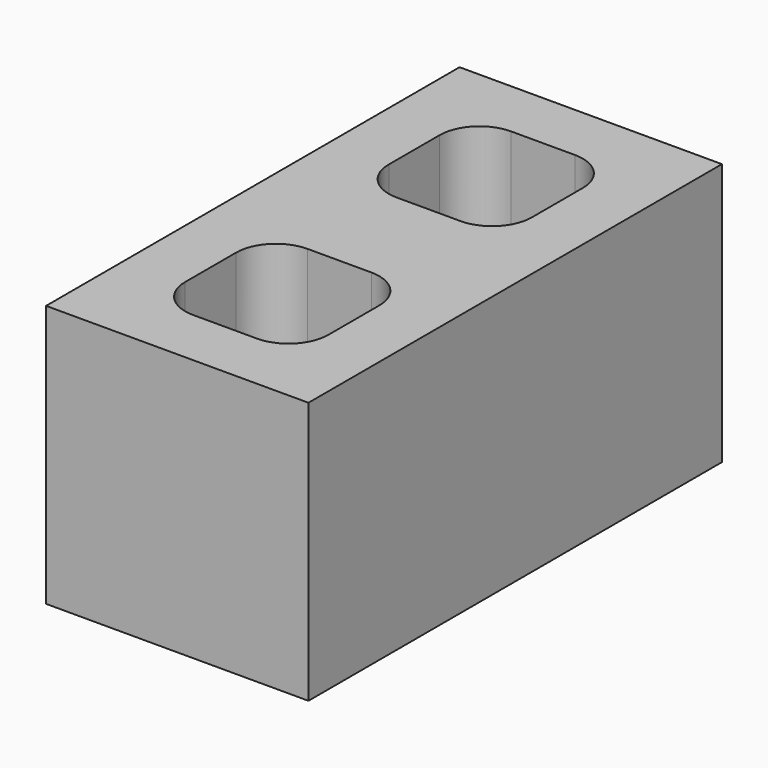
from build123d import *

# Parameters (mm, degrees)
F0_W     = 16.764
F0_H     = 33.02
F1_DEPTH = 8.382
F2_W     = 9.144
F2_H     = 9.144
F3_DEPTH = 25.4
F4_R     = 2.54


# Not quite as in the source:
# - two fillets or chamfers of one size are made in one step
# - a pattern or mirror of a feature is missing from the dataset's text; its kind, count and spacing are read off the source's solid


with BuildPart() as f1:
    # F0 (on Top) → F1 (new body, symmetric)
    with BuildSketch(Plane.XY):
        Rectangle(F0_W, F0_H)
    extrude(amount=F1_DEPTH, both=True)

    # F2 (on face) → F3 (cut)
    with BuildSketch(Plane.XY.offset(8.382)):
        with Locations((0, 8.128)):
            Rectangle(F2_W, F2_H)
    f3 = extrude(amount=-F3_DEPTH, mode=Mode.SUBTRACT)

    # F3_copies: F3 across plane
    add(f3.mirror(Plane(origin=(0, 0, 0), x_dir=(0, 0, -1), z_dir=(0, -1, 0))), mode=Mode.SUBTRACT)

    # F4
    f4_edges = [f1.edges().sort_by_distance(p)[0] for p in [
        (-4.572, 12.7, 0),
        (4.572, 12.7, 0),
        (-4.572, 3.556, 0),
        (-4.572, -12.7, 0),
        (4.572, -12.7, 0),
        (4.572, -3.556, 0),
        (-4.572, -3.556, 0),
        (4.572, 3.556, 0),
    ]]
    fillet(f4_edges, radius=F4_R)


solid = f1.part
